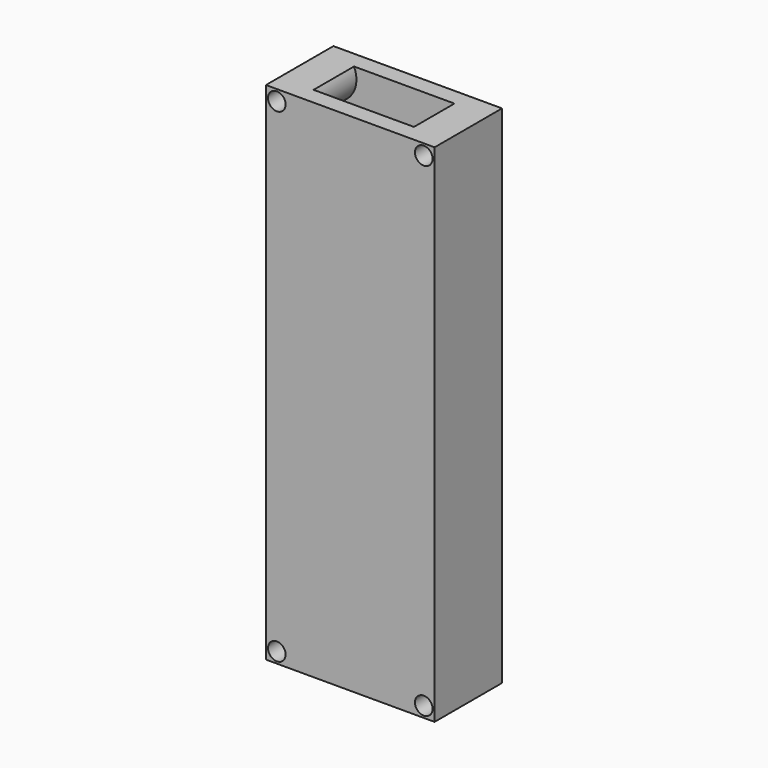
from build123d import *

# Parameters (mm, degrees)
F0_W     = 25.4
F0_H     = 76.2
F0_R     = 1.328071913
F1_DEPTH = 12.7
F2_T     = 2.54


# Not quite as in the source:
# - a shell that OpenCascade refuses in one call is made with other operations: the cavity is built on its own and cut out


with BuildPart() as f1:
    # F0 (on Front) → F1 (new body)
    with BuildSketch(Plane.XZ):
        Rectangle(F0_W, F0_H)
        with Locations((-11.0691860318, -36.4708118141)):
            Circle(F0_R, mode=Mode.SUBTRACT)
        with Locations((11.0691860318, -36.4708118141)):
            Circle(F0_R, mode=Mode.SUBTRACT)
        with Locations((-11.0691860318, 36.4708118141)):
            Circle(F0_R, mode=Mode.SUBTRACT)
        with Locations((11.0691860318, 36.4708118141)):
            Circle(F0_R, mode=Mode.SUBTRACT)
    extrude(amount=F1_DEPTH)

    # F2: shell of thickness 2.54, made by hand


with BuildPart() as f2_core1:
    # F2_t2: copy of F1
    add(f1.part)

    # the walls: a layer under each face that stays
    f2_faces = [f2_core1.faces().sort_by_distance(p)[0] for p in [
        (12.7, -6.35, 0),
        (-12.7, -6.35, 0),
        (0, -6.35, -38.1),
        (-12.3972579448, -6.35, -36.4708118141),
        (9.7411141188, -6.35, -36.4708118141),
        (-12.3972579448, -6.35, 36.4708118141),
        (9.7411141188, -6.35, 36.4708118141),
        (0, 0, 0),
        (0, -12.7, 0),
    ]]
    thicken(f2_faces, amount=-F2_T, mode=Mode.SUBTRACT)


with BuildPart() as f1_1:
    add(f1.part)

    # what is left inside the walls is the cavity
    f2_cavity = [f2_core1.part.solids().sort_by_distance(p)[0] for p in [
        (0, -2.5654, -11.006667),
    ]]
    add(f2_cavity, mode=Mode.SUBTRACT)


solid = f1_1.part
